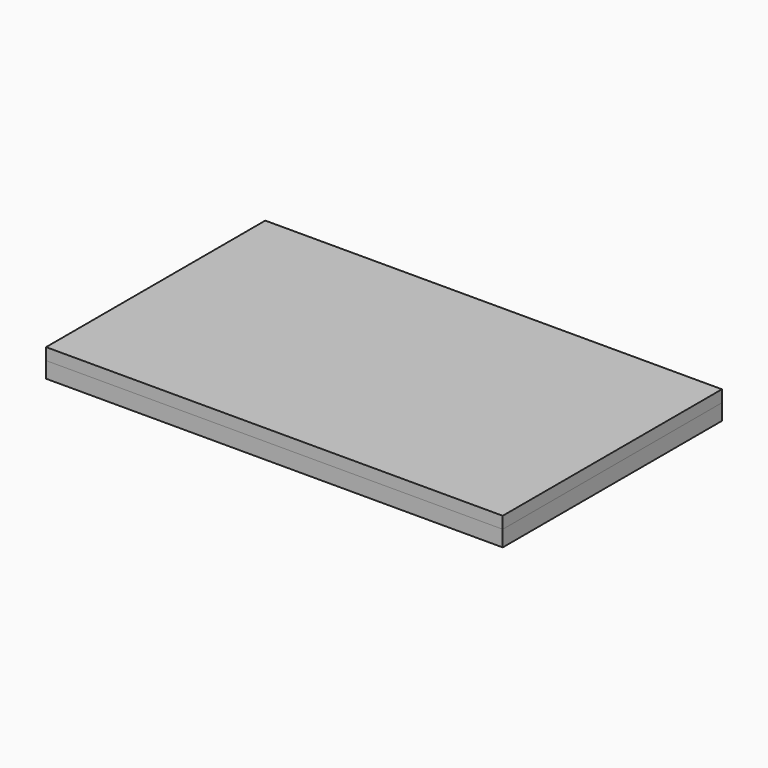
from build123d import *

# Parameters (mm, degrees)
F3_W       = 1000
F3_H       = 35
F7_DEPTH   = 35
F6_W       = 1000
F6_H       = 35
F8_DEPTH   = 35
F4_W       = 35
F4_H       = 600
F9_DEPTH   = 35
F5_W       = 35
F5_H       = 600
F10_DEPTH  = 35
F11_SIZE   = 34.99999
F12_SIZE   = 34.99999
F13_SIZE   = 34.99999
F14_SIZE   = 34.99999
F15_SIZE   = 34.99999
F15_2_SIZE = 34.99999
F16_SIZE   = 34.99999
F16_2_SIZE = 34.99999
F2_W       = 1000
F2_H       = 600
F17_DEPTH  = 26


# Not quite as in the source:
# - a fillet or chamfer is up to 0.001 mm smaller than in the source, because OpenCascade refuses the exact size


with BuildPart() as f7:
    # F3 (on Top) → F7 (new body)
    with BuildSketch(Plane.XY):
        with Locations((500, 17.5)):
            Rectangle(F3_W, F3_H)
    extrude(amount=-F7_DEPTH)

    # F14 (size 35 in the source; OpenCascade refuses exactly that, so slightly less here)
    f14_edges = [f7.edges().sort_by_distance(p)[0] for p in [
        (1000, 35, -17.5),
    ]]
    chamfer(f14_edges, length=F14_SIZE)

    # F15 (size 35 in the source; OpenCascade refuses exactly that, so slightly less here)
    f15_edges = [f7.edges().sort_by_distance(p)[0] for p in [
        (0, 35, -17.5),
    ]]
    chamfer(f15_edges, length=F15_SIZE)


with BuildPart() as f8:
    # F6 (on Top) → F8 (new body)
    with BuildSketch(Plane.XY):
        with Locations((500, 582.5)):
            Rectangle(F6_W, F6_H)
    extrude(amount=-F8_DEPTH)

    # F12 (size 35 in the source; OpenCascade refuses exactly that, so slightly less here)
    f12_edges = [f8.edges().sort_by_distance(p)[0] for p in [
        (1000, 565, -17.5),
    ]]
    chamfer(f12_edges, length=F12_SIZE)

    # F16#2 (size 35 in the source; OpenCascade refuses exactly that, so slightly less here)
    f16_2_edges = [f8.edges().sort_by_distance(p)[0] for p in [
        (0, 565, -17.5),
    ]]
    chamfer(f16_2_edges, length=F16_2_SIZE)


with BuildPart() as f9:
    # F4 (on Top) → F9 (new body)
    with BuildSketch(Plane.XY):
        with Locations((17.5, 300)):
            Rectangle(F4_W, F4_H)
    extrude(amount=-F9_DEPTH)

    # F15#2 (size 35 in the source; OpenCascade refuses exactly that, so slightly less here)
    f15_2_edges = [f9.edges().sort_by_distance(p)[0] for p in [
        (35, 0, -17.5),
    ]]
    chamfer(f15_2_edges, length=F15_2_SIZE)

    # F16 (size 35 in the source; OpenCascade refuses exactly that, so slightly less here)
    f16_edges = [f9.edges().sort_by_distance(p)[0] for p in [
        (35, 600, -17.5),
    ]]
    chamfer(f16_edges, length=F16_SIZE)


with BuildPart() as f10:
    # F5 (on Top) → F10 (new body)
    with BuildSketch(Plane.XY):
        with Locations((982.5, 300)):
            Rectangle(F5_W, F5_H)
    extrude(amount=-F10_DEPTH)

    # F11 (size 35 in the source; OpenCascade refuses exactly that, so slightly less here)
    f11_edges = [f10.edges().sort_by_distance(p)[0] for p in [
        (965, 600, -17.5),
    ]]
    chamfer(f11_edges, length=F11_SIZE)

    # F13 (size 35 in the source; OpenCascade refuses exactly that, so slightly less here)
    f13_edges = [f10.edges().sort_by_distance(p)[0] for p in [
        (965, 0, -17.5),
    ]]
    chamfer(f13_edges, length=F13_SIZE)


with BuildPart() as f17:
    # F2 (on Top) → F17 (new body)
    with BuildSketch(Plane.XY):
        with Locations((500, 300)):
            Rectangle(F2_W, F2_H)
    extrude(amount=F17_DEPTH)


solid = Compound([f7.part, f8.part, f9.part, f10.part, f17.part])
